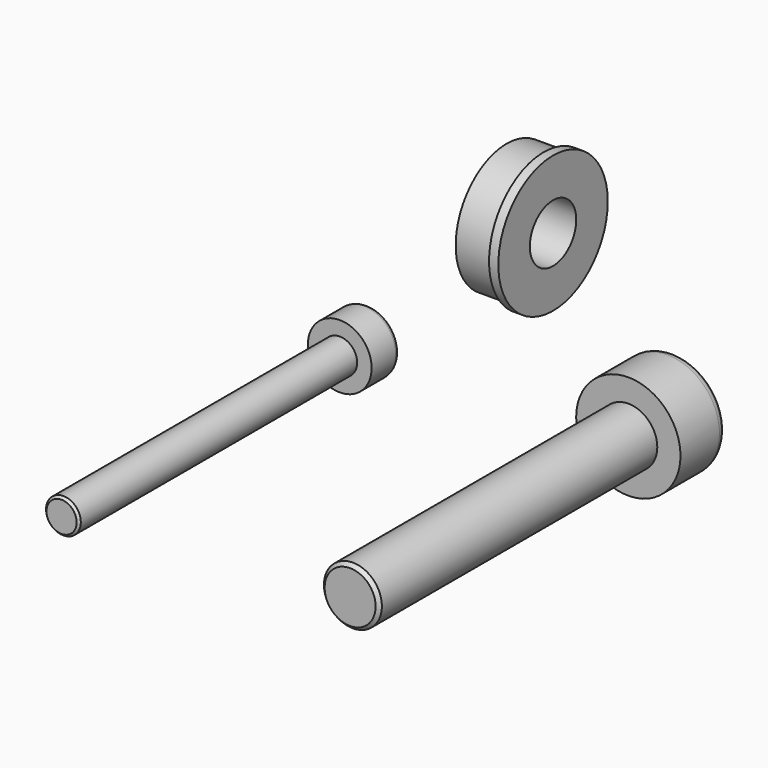
from build123d import *

# Parameters (mm, degrees)
F0_R      = 2.75
F1_DEPTH  = 3
F2_R      = 1.5
F3_DEPTH  = 30
F4_SIZE   = 0.2
F6_DEPTH  = 2
F7_R      = 0.4
F8_R      = 2.5
F9_DEPTH  = 30
F10_R     = 4.5
F10_R_2   = 2.5
F11_DEPTH = 5
F12_R     = 0.8
F13_SIZE  = 0.3
F15_DEPTH = 4


with BuildPart() as f1:
    # F0 (on Front) → F1 (new body)
    with BuildSketch(Plane.XZ):
        Circle(F0_R)
    extrude(amount=F1_DEPTH)

    # F2 (on face) → F3 (join)
    with BuildSketch(Plane.XZ.offset(3)):
        Circle(F2_R)
    extrude(amount=F3_DEPTH)

    # F4
    f4_edges = [f1.edges().sort_by_distance(p)[0] for p in [
        (-1.5, -33, 0),
    ]]
    chamfer(f4_edges, length=F4_SIZE)

    # F5 (on face) → F6 (cut)
    with BuildSketch(Plane(origin=(0, 0, 0), x_dir=(-1, 0, 0), z_dir=(0, 1, 0))):
        Polygon((1.443375673, 0), (0.7216878365, 1.25), (-0.7216878365, 1.25), (-1.443375673, 0), (-0.7216878365, -1.25), (0.7216878365, -1.25), align=None)
    extrude(amount=-F6_DEPTH, mode=Mode.SUBTRACT)

    # F7
    f7_edges = [f1.edges().sort_by_distance(p)[0] for p in [
        (-2.75, 0, 0),
    ]]
    fillet(f7_edges, radius=F7_R)


with BuildPart() as f9:
    # F8 (on Front) → F9 (new body)
    with BuildSketch(Plane.XZ):
        with Locations((22.4943347275, 0)):
            Circle(F8_R)
    extrude(amount=F9_DEPTH)

    # F10 (on face) → F11 (join)
    with BuildSketch(Plane(origin=(0, 0, 0), x_dir=(-1, 0, 0), z_dir=(0, 1, 0))):
        with Locations((-22.4943347275, 0)):
            Circle(F10_R)
        with Locations((-22.4943347275, 0)):
            Circle(F10_R_2, mode=Mode.SUBTRACT)
        with Locations((-22.4943347275, 0)):
            Circle(F10_R_2)
    extrude(amount=F11_DEPTH)

    # F12
    f12_edges = [f9.edges().sort_by_distance(p)[0] for p in [
        (26.994335, 5, 0),
    ]]
    fillet(f12_edges, radius=F12_R)

    # F13
    f13_edges = [f9.edges().sort_by_distance(p)[0] for p in [
        (19.994335, -30, 0),
    ]]
    chamfer(f13_edges, length=F13_SIZE)

    # F14 (on face) → F15 (cut)
    with BuildSketch(Plane(origin=(0, 5, 0), x_dir=(-1, 0, 0), z_dir=(0, 1, 0))):
        Polygon((-23.6490352659, -2), (-21.3396341891, -2), (-20.1849336508, 0), (-21.3396341891, 2), (-23.6490352659, 2), (-24.8037358043, 0), align=None)
    extrude(amount=-F15_DEPTH, mode=Mode.SUBTRACT)


with BuildPart() as f17:
    # F16 (on Top) → F17 (revolve)
    with BuildSketch(Plane.XY):
        Polygon((0, 22.5), (0, 25.9), (-0.8, 25.9), (-0.8, 25.5), (-4, 25.5), (-4, 22.5), align=None)
    revolve(axis=Axis((-6.1384743312, 20, 0), (-1, 0, 0)))


solid = Compound([f1.part, f9.part, f17.part])
